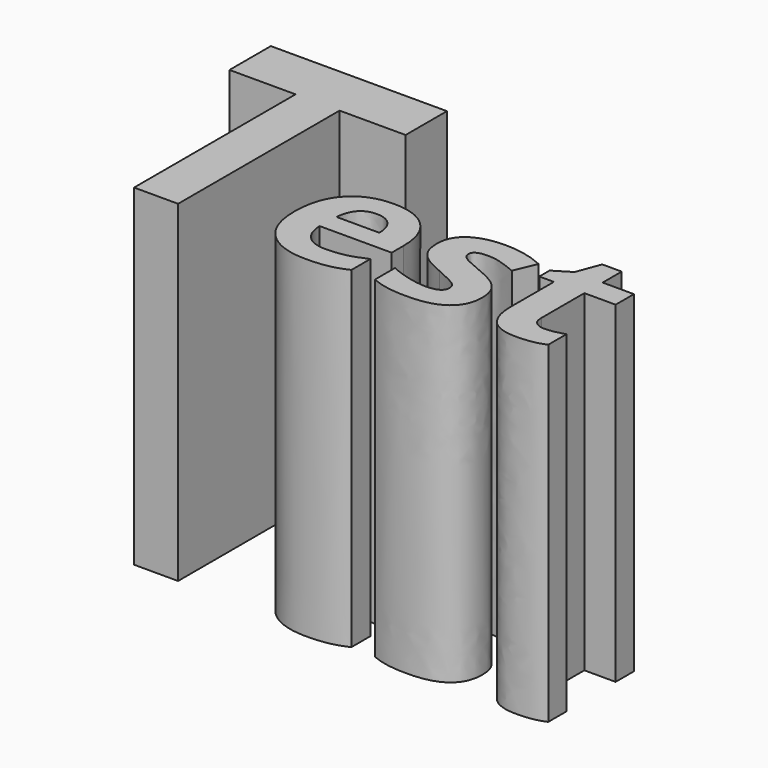
from build123d import *

# Parameters (mm, degrees)
F0_TEXT_SIZE = 46.9499319378
F1_DEPTH     = 76.2


# Not quite as in the source:
# - Text() gives the source's letters only with a copy of the font that has no kerning and outlines rounded to 1/6400 em; it was checked with that copy


with BuildPart() as f1:
    # F0 (on Top) → F1 (new body)
    with BuildSketch(Plane.XY):
        Polygon((-67.3883929849, 25.1334570348), (-52.2313377711, 25.1334570348), (-52.2313377711, -21.1823452264), (-42.1340539012, -21.1823452264), (-42.1340539012, 25.1334570348), (-26.9769986874, 25.1334570348), (-26.9769986874, 36.9867905974), (-67.3883929849, 36.9867905974), align=None)
        with Locations((-26.1212345213, -23.1579020619)):
            Text('est', F0_TEXT_SIZE, font='Open Sans', font_style=FontStyle.BOLD, text_align=(TextAlign.LEFT, TextAlign.BOTTOM))
    extrude(amount=F1_DEPTH)


solid = f1.part
